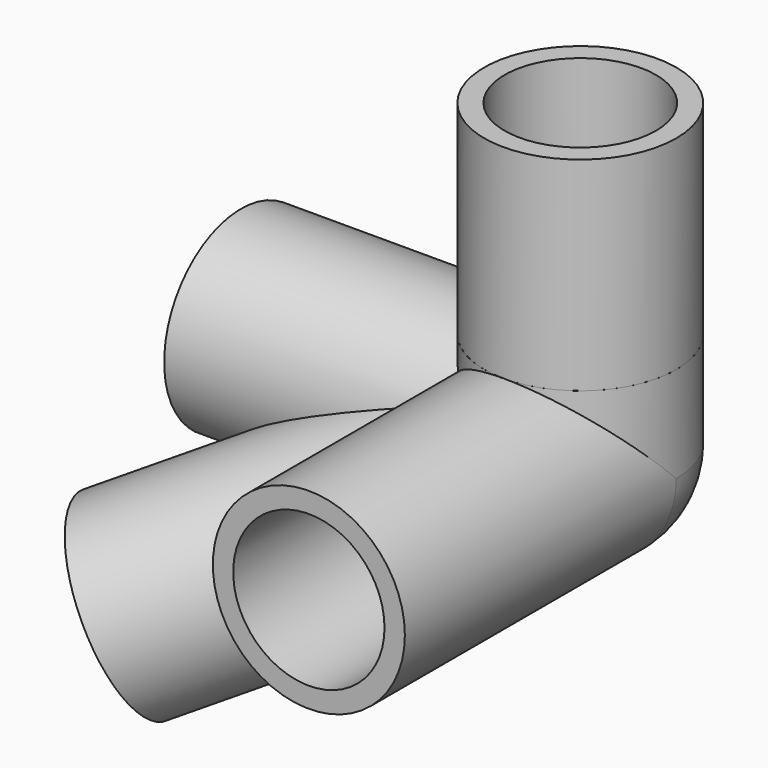
from build123d import *

# Parameters (mm, degrees)
F0_R      = 14.15
F0_R_2    = 11.15
F1_DEPTH  = 25
F2_R      = 14.15
F3_DEPTH  = 5
F4_R      = 14.15
F4_R_2    = 11.15
F5_DEPTH  = 50
F6_R      = 14.15
F6_R_2    = 11.15
F7_DEPTH  = 50
F16_R     = 14.15
F16_R_2   = 11.15
F17_DEPTH = 30
F10_R     = 11.15
F18_DEPTH = 35
F11_R     = 11.15
F19_DEPTH = 30
F20_R     = 11.15
F21_DEPTH = 50
F22_R     = 11.15
F23_DEPTH = 25
F24_R     = 11.15
F25_DEPTH = 50.1
F26_R     = 11.15
F27_DEPTH = 25


with BuildPart() as f1:
    # F0 (on Top) → F1 (new body)
    with BuildSketch(Plane.XY):
        Circle(F0_R)
        Circle(F0_R_2, mode=Mode.SUBTRACT)
    extrude(amount=F1_DEPTH)

    # F2 (on Top) → F3 (join)
    with BuildSketch(Plane.XY):
        Circle(F2_R)
    extrude(amount=-F3_DEPTH)


with BuildPart() as f5:
    # F4 (on Right) → F5 (new body)
    with BuildSketch(Plane.YZ):
        with Locations((0, -19.15)):
            Circle(F4_R)
        with Locations((0, -19.15)):
            Circle(F4_R_2, mode=Mode.SUBTRACT)
    extrude(amount=-F5_DEPTH)

    # F6 (on Front) → F7 (join)
    with BuildSketch(Plane.XZ):
        with Locations((0, -19.15)):
            Circle(F6_R)
        with Locations((0, -19.15)):
            Circle(F6_R_2, mode=Mode.SUBTRACT)
    extrude(amount=F7_DEPTH)

    # F8 (on face) → F9 (revolve)
    with BuildSketch(Plane(origin=(0, 0, 0), x_dir=(-1, 0, 0), z_dir=(0, 1, 0))):
        with BuildLine():
            Line((-14.15, -5), (-14.15, -19.15))
            ThreePointArc((-14.15, -19.15), (-10.0055609538, -29.1555609538), (0, -33.3))
            Line((0, -33.3), (0, -5))
            Line((0, -5), (-14.15, -5))
        make_face()
    revolve(axis=Axis((0, 0, -19.15), (0, 0, 1)))

    # F16 (on line) → F17 (join, symmetric)
    with BuildSketch(Plane(origin=(-30.8408370839, -15.4439407788, -17.2721216794), x_dir=(0.3493154192, -0.9163554539, 0.1956308258), z_dir=(-0.7995117993, -0.4003656855, -0.4477590878))):
        with Locations((-3.7478874438, -16.7074557394)):
            Circle(F16_R)
        with Locations((-3.7478874438, -16.7074557394)):
            Circle(F16_R_2, mode=Mode.SUBTRACT)
    extrude(amount=F17_DEPTH, both=True)

    # F10 (on face) → F18 (cut)
    with BuildSketch(Plane(origin=(-50, 0, 0), x_dir=(0, -1, 0), z_dir=(-1, 0, 0))):
        with Locations((0, -19.15)):
            Circle(F10_R)
    extrude(amount=-F18_DEPTH, mode=Mode.SUBTRACT)

    # F11 (on face) → F19 (cut)
    with BuildSketch(Plane.XZ.offset(50)):
        with Locations((0, -19.15)):
            Circle(F11_R)
    extrude(amount=-F19_DEPTH, mode=Mode.SUBTRACT)

    # F20 (on face) → F21 (join)
    with BuildSketch(Plane(origin=(-50, 0, 0), x_dir=(0, -1, 0), z_dir=(-1, 0, 0))):
        with Locations((0, -19.15)):
            Circle(F20_R)
    extrude(amount=-F21_DEPTH)

    # F22 (on face) → F23 (cut)
    with BuildSketch(Plane(origin=(-50, 0, 0), x_dir=(0, -1, 0), z_dir=(-1, 0, 0))):
        with Locations((0, -19.15)):
            Circle(F22_R)
    extrude(amount=-F23_DEPTH, mode=Mode.SUBTRACT)

    # F24 (on face) → F25 (join)
    with BuildSketch(Plane.XZ.offset(50)):
        with Locations((0, -19.15)):
            Circle(F24_R)
    extrude(amount=-F25_DEPTH)

    # F26 (on face) → F27 (cut)
    with BuildSketch(Plane.XZ.offset(50)):
        with Locations((0, -19.15)):
            Circle(F26_R)
    extrude(amount=-F27_DEPTH, mode=Mode.SUBTRACT)


solid = Compound([f1.part, f5.part])
